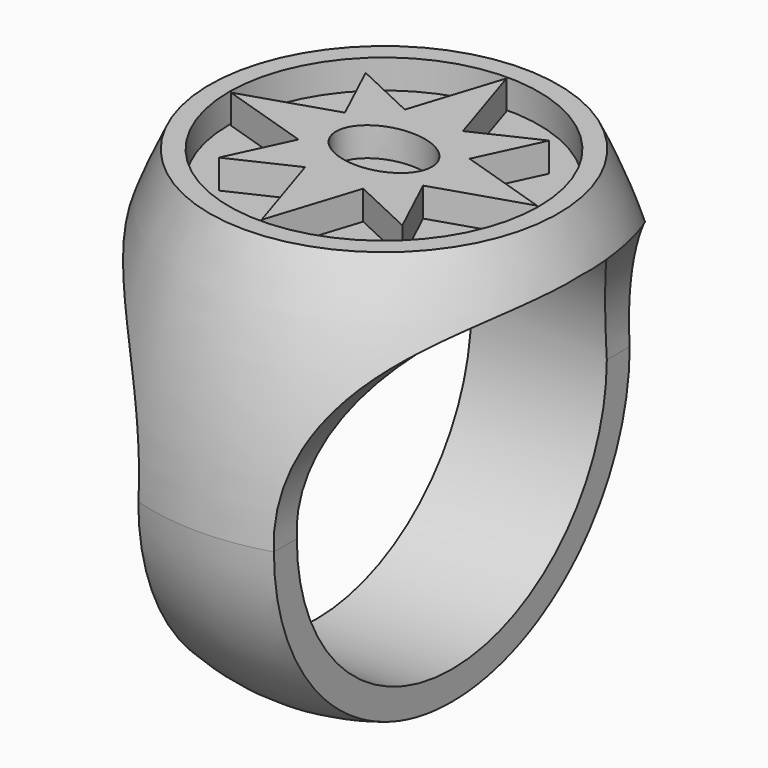
from build123d import *

# Parameters (mm, degrees)
F2_R     = 10
F3_DEPTH = 12.5
F5_DEPTH = 12.5
F6_R     = 8
F7_DEPTH = 1.5


# Not quite as in the source:
# - a feature of the source that left no trace in its solid (it failed there, or was rolled back) is left out


with BuildPart() as f1:
    # F0 (on Right) → F1 (revolve)
    with BuildSketch(Plane.YZ):
        with BuildLine():
            Line((0, -24.5), (0, 0))
            Line((0, 0), (-9, 0))
            ThreePointArc((-9, 0), (-11.177394056, -6.0874254266), (-12, -12.5))
            ThreePointArc((-12, -12.5), (-8.4852813742, -20.9852813742), (0, -24.5))
        make_face()
    revolve(axis=Axis((0, 0, -12.25), (0, 0, -1)))

    # F2 (on Right) → F3 (cut, symmetric)
    with BuildSketch(Plane.YZ):
        with Locations((0, -12.5)):
            Circle(F2_R)
    extrude(amount=F3_DEPTH, both=True, mode=Mode.SUBTRACT)

    # F4 (on Front) → F5 (cut, symmetric)
    with BuildSketch(Plane.XZ):
        with BuildLine():
            Line((3.5, -12.5), (3.5, -26.5))
            Line((3.5, -26.5), (11.6508146748, -26.5))
            Line((11.6508146748, -26.5), (11.6508146748, -2.5))
            Line((11.6508146748, -2.5), (10.1532964036, -2.5))
            ThreePointArc((10.1532964036, -2.5), (5.1580549578, -6.3898354571), (3.5, -12.5))
        make_face()
        with BuildLine():
            Line((-11.6508146748, -26.5), (-3.5, -26.5))
            Line((-3.5, -26.5), (-3.5, -12.5))
            ThreePointArc((-3.5, -12.5), (-5.1580549578, -6.3898354571), (-10.1532964036, -2.5))
            Line((-10.1532964036, -2.5), (-11.6508146748, -2.5))
            Line((-11.6508146748, -2.5), (-11.6508146748, -26.5))
        make_face()
    extrude(amount=F5_DEPTH, both=True, mode=Mode.SUBTRACT)

    # F6 (on face) → F7 (cut)
    with BuildSketch(Plane.XY):
        Circle(F6_R)
        Polygon((3.2175301086, 1.5), (7.9, 0), (3.2175301086, -1.5), (4.7363741323, -4.7363741323), (1.5, -3.2175301086), (0, -7.9), (-1.5, -3.2175301086), (-4.7363741323, -4.7363741323), (-3.2175301086, -1.5), (-7.9, 0), (-3.2175301086, 1.5), (-4.7363741323, 4.7363741323), (-1.5, 3.2175301086), (0, 7.9), (1.5, 3.2175301086), (4.7363741323, 4.7363741323), align=None, mode=Mode.SUBTRACT)
        with BuildLine():
            add(Edge.make_bspline(
                [(2.4737748317, 0), (2.4737748317, 3.1158306041), (-1.2368874159, 1.557915302), (-4.9475496635, 0), (-1.2368874159, -1.557915302), (2.4737748317, -3.1158306041), (2.4737748317, 0)],
                knots=[0, 0, 0, 2.0943951024, 2.0943951024, 4.1887902048, 4.1887902048, 6.2831853072, 6.2831853072, 6.2831853072], degree=2, weights=[1, 0.5, 1, 0.5, 1, 0.5, 1]))
        make_face()
    extrude(amount=-F7_DEPTH, mode=Mode.SUBTRACT)


solid = f1.part
